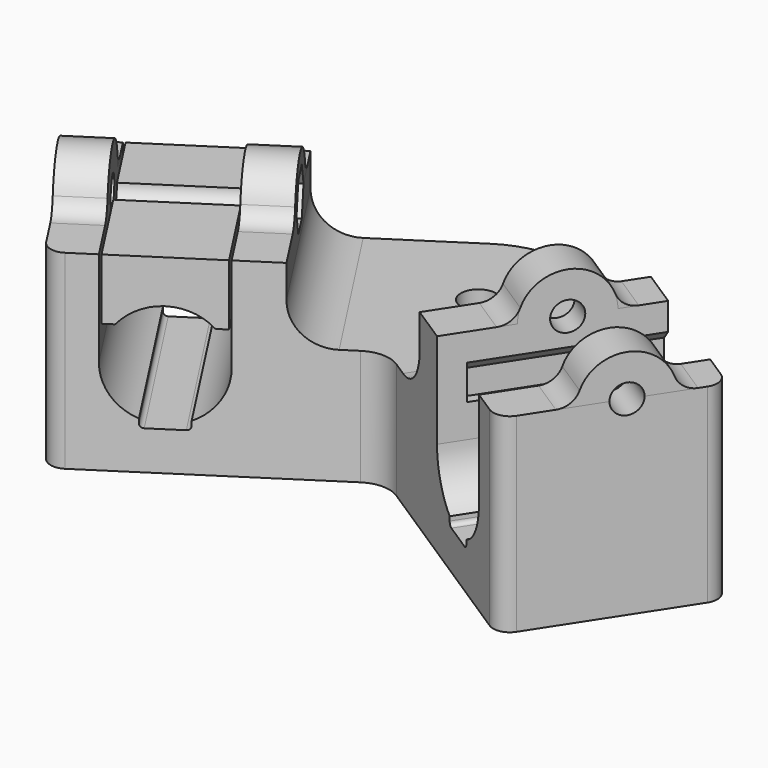
from build123d import *

# Parameters (mm, degrees)
F1_DEPTH      = 23
F7_DEPTH      = 18
F8_R          = 10
F10_DEPTH     = 46
F9_R          = 10
F11_DEPTH     = 46
F14_DEPTH     = 33.001
F15_DEPTH     = 33.001
F16_R         = 8
F17_R         = 10
F20_DEPTH     = 40
F21_DEPTH     = 40
F24_DEPTH     = 46
F25_DEPTH     = 46
F26_T1_DEPTH  = 10.4
F26_T3_DEPTH  = 10.4
F26_T5_DEPTH  = 10.4
F26_T7_DEPTH  = 10.4
F26_T9_DEPTH  = 10.4
F26_T11_DEPTH = 10.4
F26_T13_DEPTH = 10.4
F26_T15_DEPTH = 10.4
F27_R         = 4.25
F27_W         = 2
F27_H         = 2
F28_DEPTH     = 28
F30_DEPTH     = 46
F31_R         = 3.5
F32_DEPTH     = 46
F33_R         = 3.5
F34_DEPTH     = 46
F36_DEPTH     = 4
F38_DEPTH     = 4
F39_R         = 4
F40_W         = 6
F40_H         = 8.2964466094
F41_DEPTH     = 2.4
F42_W         = 6.0000000001
F42_H         = 8.2964466094
F43_DEPTH     = 2.4


# Not quite as in the source:
# - a fillet or chamfer that OpenCascade refuses, or shapes differently, is made with other operations: its cross-section is extruded or revolved along the edge and cut away or added


with BuildPart() as f1:
    # F0 (on Top) → F1 (new body, symmetric)
    with BuildSketch(Plane.XY):
        with BuildLine():
            Line((-79.7443559494, 80.5657352366), (-54.6909603387, 41.9868891111))
            Line((-54.6909603387, 41.9868891111), (0, 77.5036140343))
            Line((0, 77.5036140343), (54.6909603387, 41.9868891111))
            Line((54.6909603387, 41.9868891111), (79.7443559494, 80.5657352366))
            Line((79.7443559494, 80.5657352366), (12.5266978053, 124.2173928323))
            ThreePointArc((12.5266978053, 124.2173928323), (6.5323529282, 126.9808236715), (0, 127.9279697696))
            ThreePointArc((0, 127.9279697696), (-6.5323529282, 126.9808236715), (-12.5266978053, 124.2173928323))
            Line((-12.5266978053, 124.2173928323), (-79.7443559494, 80.5657352366))
        make_face()
    extrude(amount=F1_DEPTH, both=True)

    # F2 (on Top) → F4 (revolve, cut)
    with BuildSketch(Plane.XY):
        Polygon((-71.0221820428, 86.2299812008), (-45.9687864321, 47.6511350753), (-35.401537276, 54.5135869165), (-60.4549328867, 93.0924330419), align=None)
    revolve(axis=Axis((-28.5739341007, 44, 0), (-0.544639035, 0.8386705679, 0)), mode=Mode.SUBTRACT)

    # F3 (on Top) → F5 (revolve, cut)
    with BuildSketch(Plane.XY):
        Polygon((49.8876837306, 99.9548848831), (24.8342881199, 61.3760387576), (35.401537276, 54.5135869165), (60.4549328867, 93.0924330419), align=None)
    revolve(axis=Axis((28.5739341007, 44, 0), (0.544639035, 0.8386705679, 0)), mode=Mode.SUBTRACT)

    # F6 (on face) → F7 (cut)
    with BuildSketch(Plane.XY.offset(23)):
        with BuildLine():
            Line((-12.5266978053, 124.2173928323), (-41.1655098239, 105.6191308473))
            Line((-41.1655098239, 105.6191308473), (-16.1121142132, 67.0402847218))
            Line((-16.1121142132, 67.0402847218), (0, 77.5036140343))
            Line((0, 77.5036140343), (16.1121142132, 67.0402847218))
            Line((16.1121142132, 67.0402847218), (41.1655098239, 105.6191308473))
            Line((41.1655098239, 105.6191308473), (12.5266978053, 124.2173928323))
            ThreePointArc((12.5266978053, 124.2173928323), (6.5323529282, 126.9808236715), (0, 127.9279697696))
            ThreePointArc((0, 127.9279697696), (-6.5323529282, 126.9808236715), (-12.5266978053, 124.2173928323))
        make_face()
    extrude(amount=-F7_DEPTH, mode=Mode.SUBTRACT)

    # F8 (on face) → F10 (join, through all)
    with BuildSketch(Plane(origin=(-19.2894230627, -12.5266978053, 0), x_dir=(0.544639035, -0.8386705679, 0), z_dir=(-0.8386705679, -0.544639035, 0))):
        with Locations((-91, 23)):
            Circle(F8_R)
    extrude(amount=-F10_DEPTH)

    # F9 (on face) → F11 (join, through all)
    with BuildSketch(Plane(origin=(19.2894230627, -12.5266978053, 0), x_dir=(0.544639035, 0.8386705679, 0), z_dir=(0.8386705679, -0.544639035, 0))):
        with Locations((91, 23)):
            Circle(F9_R)
    extrude(amount=-F11_DEPTH)

    # F12 (on Top) → F14 (cut, through all)
    with BuildSketch(Plane.XY):
        Polygon((-71.0221820428, 86.2299812008), (-45.9687864321, 47.6511350753), (-35.401537276, 54.5135869165), (-24.8342881199, 61.3760387576), (-49.8876837306, 99.9548848831), (-60.4549328867, 93.0924330419), align=None)
    extrude(amount=F14_DEPTH, mode=Mode.SUBTRACT)

    # F13 (on Top) → F15 (cut, through all)
    with BuildSketch(Plane.XY):
        Polygon((24.8342881199, 61.3760387576), (35.401537276, 54.5135869165), (45.9687864321, 47.6511350753), (71.0221820428, 86.2299812008), (60.4549328867, 93.0924330419), (49.8876837306, 99.9548848831), align=None)
    extrude(amount=F15_DEPTH, mode=Mode.SUBTRACT)

    # F16
    f16_edges = [f1.edges().sort_by_distance(p)[0] for p in [
        (0, 77.503614, 2.5),
        (0, 77.503614, -11.5),
    ]]
    fillet(f16_edges, radius=F16_R)

    # F17
    f17_edges = [f1.edges().sort_by_distance(p)[0] for p in [
        (28.638812, 86.329708, 5),
        (-28.638812, 86.329708, 5),
    ]]
    fillet(f17_edges, radius=F17_R)

    # F18 (on face) → F20 (cut)
    with BuildSketch(Plane(origin=(-60.4549328867, 93.0924330419, 0), x_dir=(-0.8386705679, -0.544639035, 0), z_dir=(-0.544639035, 0.8386705679, 0))):
        Polygon((12.6, 16.4), (-12.6, 16.4), (-15, 14), (-15, 8), (15, 8), (15, 14), align=None)
    extrude(amount=-F20_DEPTH, mode=Mode.SUBTRACT)

    # F19 (on face) → F21 (cut)
    with BuildSketch(Plane(origin=(60.4549328867, 93.0924330419, 0), x_dir=(-0.8386705679, 0.544639035, 0), z_dir=(0.544639035, 0.8386705679, 0))):
        Polygon((-15, 14), (-15, 8), (15, 8), (15, 14), (12.6, 16.4), (-12.6, 16.4), align=None)
    extrude(amount=-F21_DEPTH, mode=Mode.SUBTRACT)

    # F22 (on face) → F24 (cut, through all)
    with BuildSketch(Plane(origin=(-60.4549328867, 93.0924330419, 0), x_dir=(-0.8386705679, -0.544639035, 0), z_dir=(-0.544639035, 0.8386705679, 0))):
        with BuildLine():
            Line((5, -10.6), (-5, -10.6))
            Line((-5, -10.6), (-5, -12.6))
            ThreePointArc((-5, -12.6), (-4.7071067812, -13.3071067812), (-4, -13.6))
            Line((-4, -13.6), (4, -13.6))
            ThreePointArc((4, -13.6), (4.7071067812, -13.3071067812), (5, -12.6))
            Line((5, -12.6), (5, -10.6))
        make_face()
    extrude(amount=-F24_DEPTH, mode=Mode.SUBTRACT)

    # F23 (on face) → F25 (cut, through all)
    with BuildSketch(Plane(origin=(60.4549328867, 93.0924330419, 0), x_dir=(-0.8386705679, 0.544639035, 0), z_dir=(0.544639035, 0.8386705679, 0))):
        with BuildLine():
            ThreePointArc((-5, -12.6), (-4.7071067812, -13.3071067812), (-4, -13.6))
            Line((-4, -13.6), (4, -13.6))
            ThreePointArc((4, -13.6), (4.7071067812, -13.3071067812), (5, -12.6))
            Line((5, -12.6), (5, -10.6))
            Line((5, -10.6), (-5, -10.6))
            Line((-5, -10.6), (-5, -12.6))
        make_face()
    extrude(amount=-F25_DEPTH, mode=Mode.SUBTRACT)

    # F26: fillet of radius 5 on 8 edges, made by hand

    # F26_s2 → F26_t1 (join)
    with BuildSketch(Plane(origin=(10.5672491561, 6.8624518412, 0), x_dir=(0, 0, 1), z_dir=(0.8386705679, 0.544639035, 0))):
        with BuildLine():
            ThreePointArc((23, -76.8578643763), (23.9175170954, -79.7446157222), (26.3333333333, -81.5719095842))
            ThreePointArc((26.3333333333, -81.5719095842), (24.6910197873, -81.1440144035), (23, -81))
            Line((23, -81), (23, -76.8578643763))
        make_face()
    extrude(amount=F26_T1_DEPTH)

    # F26_s4 → F26_t3 (join)
    with BuildSketch(Plane(origin=(-19.2894230627, -12.5266978053, 0), x_dir=(0, 0, 1), z_dir=(0.8386705679, 0.544639035, 0))):
        with BuildLine():
            ThreePointArc((23, -76.8578643763), (23.9175170954, -79.7446157222), (26.3333333333, -81.5719095842))
            ThreePointArc((26.3333333333, -81.5719095842), (24.6910197873, -81.1440144035), (23, -81))
            Line((23, -81), (23, -76.8578643763))
        make_face()
    extrude(amount=F26_T3_DEPTH)

    # F26_s6 → F26_t5 (join)
    with BuildSketch(Plane(origin=(10.5672491561, -6.8624518412, 0), x_dir=(0, 0, 1), z_dir=(0.8386705679, -0.544639035, 0))):
        with BuildLine():
            ThreePointArc((23, -76.8578643763), (23.9175170954, -79.7446157222), (26.3333333333, -81.5719095842))
            ThreePointArc((26.3333333333, -81.5719095842), (24.6910197873, -81.1440144035), (23, -81))
            Line((23, -81), (23, -76.8578643763))
        make_face()
    extrude(amount=F26_T5_DEPTH)

    # F26_s8 → F26_t7 (join)
    with BuildSketch(Plane(origin=(-19.2894230627, 12.5266978053, 0), x_dir=(0, 0, 1), z_dir=(0.8386705679, -0.544639035, 0))):
        with BuildLine():
            ThreePointArc((23, -76.8578643763), (23.9175170954, -79.7446157222), (26.3333333333, -81.5719095842))
            ThreePointArc((26.3333333333, -81.5719095842), (24.6910197873, -81.1440144035), (23, -81))
            Line((23, -81), (23, -76.8578643763))
        make_face()
    extrude(amount=F26_T7_DEPTH)

    # F26_s10 → F26_t9 (join)
    with BuildSketch(Plane(origin=(19.2894230627, 12.5266978053, 0), x_dir=(0, 0, 1), z_dir=(-0.8386705679, -0.544639035, 0))):
        with BuildLine():
            ThreePointArc((23, 105.1421356237), (23.9175170954, 102.2553842778), (26.3333333333, 100.4280904158))
            ThreePointArc((26.3333333333, 100.4280904158), (24.6910197873, 100.8559855965), (23, 101))
            Line((23, 101), (23, 105.1421356237))
        make_face()
    extrude(amount=F26_T9_DEPTH)

    # F26_s12 → F26_t11 (join)
    with BuildSketch(Plane(origin=(-10.5672491561, -6.8624518412, 0), x_dir=(0, 0, 1), z_dir=(-0.8386705679, -0.544639035, 0))):
        with BuildLine():
            ThreePointArc((23, 105.1421356237), (23.9175170954, 102.2553842778), (26.3333333333, 100.4280904158))
            ThreePointArc((26.3333333333, 100.4280904158), (24.6910197873, 100.8559855965), (23, 101))
            Line((23, 101), (23, 105.1421356237))
        make_face()
    extrude(amount=F26_T11_DEPTH)

    # F26_s14 → F26_t13 (join)
    with BuildSketch(Plane(origin=(-10.5672491561, 6.8624518412, 0), x_dir=(0, 0, 1), z_dir=(-0.8386705679, 0.544639035, 0))):
        with BuildLine():
            ThreePointArc((23, 105.1421356237), (23.9175170954, 102.2553842778), (26.3333333333, 100.4280904158))
            ThreePointArc((26.3333333333, 100.4280904158), (24.6910197873, 100.8559855965), (23, 101))
            Line((23, 101), (23, 105.1421356237))
        make_face()
    extrude(amount=F26_T13_DEPTH)

    # F26_s16 → F26_t15 (join)
    with BuildSketch(Plane(origin=(19.2894230627, -12.5266978053, 0), x_dir=(0, 0, 1), z_dir=(-0.8386705679, 0.544639035, 0))):
        with BuildLine():
            ThreePointArc((23, 105.1421356237), (23.9175170954, 102.2553842778), (26.3333333333, 100.4280904158))
            ThreePointArc((26.3333333333, 100.4280904158), (24.6910197873, 100.8559855965), (23, 101))
            Line((23, 101), (23, 105.1421356237))
        make_face()
    extrude(amount=F26_T15_DEPTH)

    # F27 (on face) → F28 (cut, through all)
    with BuildSketch(Plane.XY.offset(5)):
        with Locations((0, 104.9279697696)):
            Circle(F27_R)
        with Locations((0, 127.9279697696)):
            Rectangle(F27_W, F27_H)
    extrude(amount=-F28_DEPTH, mode=Mode.SUBTRACT)


with BuildPart() as f30:
    # F29 (on face) → F30 (new body, through all)
    with BuildSketch(Plane(origin=(-60.4549328867, 93.0924330419, 0), x_dir=(-0.8386705679, -0.544639035, 0), z_dir=(-0.544639035, 0.8386705679, 0))):
        with BuildLine():
            ThreePointArc((-9.5235235076, 8.25), (-5.23497851, 11.4610208969), (0, 12.6))
            ThreePointArc((0, 12.6), (5.23497851, 11.4610208969), (9.5235235076, 8.25))
            Line((9.5235235076, 8.25), (14.5, 8.25))
            Line((14.5, 8.25), (14.5, 14.1464466094))
            Line((14.5, 14.1464466094), (12.1, 16.5464466094))
            Line((12.1, 16.5464466094), (12.1, 23))
            Line((12.1, 23), (0, 23))
            Line((0, 23), (-12.1, 23))
            Line((-12.1, 23), (-12.1, 16.5464466094))
            Line((-12.1, 16.5464466094), (-14.5, 14.1464466094))
            Line((-14.5, 14.1464466094), (-14.5, 8.25))
            Line((-14.5, 8.25), (-9.5235235076, 8.25))
        make_face()
    extrude(amount=-F30_DEPTH)


with BuildPart() as f32_tool:
    # F31 (on face) → F32 (new body, through all)
    with BuildSketch(Plane(origin=(-19.2894230627, -12.5266978053, 0), x_dir=(0.544639035, -0.8386705679, 0), z_dir=(-0.8386705679, -0.544639035, 0))):
        with Locations((-91, 23)):
            Circle(F31_R)
    extrude(amount=-F32_DEPTH)


with BuildPart() as f1_1:
    add(f1.part)

    # F32: cut by f32_tool
    add(f32_tool.part, mode=Mode.SUBTRACT)

    # F33 (on face) → F34 (cut, through all)
    with BuildSketch(Plane(origin=(19.2894230627, -12.5266978053, 0), x_dir=(0.544639035, 0.8386705679, 0), z_dir=(0.8386705679, -0.544639035, 0))):
        with Locations((91, 23)):
            Circle(F33_R)
    extrude(amount=-F34_DEPTH, mode=Mode.SUBTRACT)

    # F35 (on face) → F36 (cut)
    with BuildSketch(Plane(origin=(19.2894230627, 12.5266978053, 0), x_dir=(-0.544639035, 0.8386705679, 0), z_dir=(0.8386705679, 0.544639035, 0))):
        Polygon((87.6802359521, 28.75), (84.3604719042, 23), (87.6802359521, 17.25), (94.3197640477, 17.25), (97.6395280956, 23), (94.3197640477, 28.75), align=None)
    extrude(amount=-F36_DEPTH, mode=Mode.SUBTRACT)

    # F37 (on face) → F38 (cut)
    with BuildSketch(Plane(origin=(-19.2894230627, 12.5266978053, 0), x_dir=(-0.544639035, -0.8386705679, 0), z_dir=(-0.8386705679, 0.544639035, 0))):
        Polygon((-94.319764048, 28.75), (-97.6395280959, 23), (-94.319764048, 17.25), (-87.6802359523, 17.25), (-84.3604719045, 23), (-87.6802359523, 28.75), align=None)
    extrude(amount=-F38_DEPTH, mode=Mode.SUBTRACT)

    # F39
    f39_edges = [f1_1.edges().sort_by_distance(p)[0] for p in [
        (79.744356, 80.565735, 0),
        (54.69096, 41.986889, 0),
        (-54.69096, 41.986889, 0),
        (-79.744356, 80.565735, 0),
    ]]
    fillet(f39_edges, radius=F39_R)


with BuildPart() as f30_1:
    add(f30.part)

    # F32: cut by f32_tool
    add(f32_tool.part, mode=Mode.SUBTRACT)

    # F40 (on face) → F41 (cut, through all)
    with BuildSketch(Plane(origin=(-12.1607232352, -7.8972660077, 0), x_dir=(0.544639035, -0.8386705679, 0), z_dir=(-0.8386705679, -0.544639035, 0))):
        with Locations((-67.9999999999, 12.3982233047)):
            Rectangle(F40_W, F40_H)
    extrude(amount=-F41_DEPTH, mode=Mode.SUBTRACT)

    # F42 (on face) → F43 (cut, through all)
    with BuildSketch(Plane(origin=(12.1607232352, 7.8972660077, 0), x_dir=(-0.544639035, 0.8386705679, 0), z_dir=(0.8386705679, 0.544639035, 0))):
        with Locations((67.9999999999, 12.3982233047)):
            Rectangle(F42_W, F42_H)
    extrude(amount=-F43_DEPTH, mode=Mode.SUBTRACT)


solid = Compound([f1_1.part, f30_1.part])
